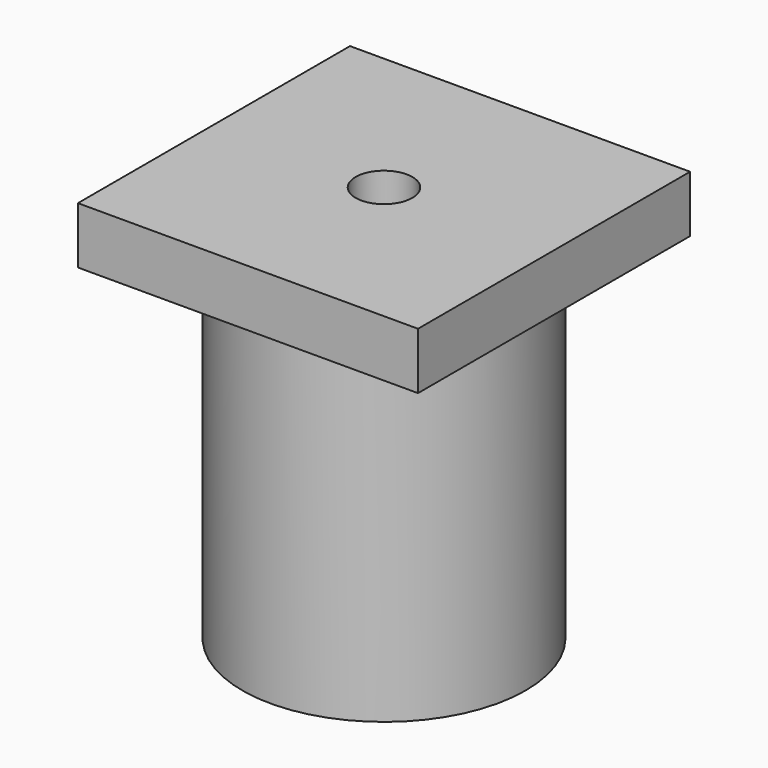
from build123d import *

# Parameters (mm, degrees)
F0_W     = 30
F0_H     = 30
F1_DEPTH = 35
F2_DEPTH = 30
F3_R     = 2.5
F4_DEPTH = 35.001
F5_W     = 30
F5_H     = 30
F5_R     = 12.5
F6_DEPTH = 30


with BuildPart() as f1:
    # F0 (on Top) → F1 (new body)
    with BuildSketch(Plane.XY):
        Rectangle(F0_W, F0_H)
        with BuildLine():
            ThreePointArc((-2.5, -6.5383484153), (-3.9686269666, 5.7662812973), (7, 0))
            ThreePointArc((7, 0), (5.7662812973, -3.9686269666), (2.5, -6.5383484153))
            Line((2.5, -6.5383484153), (2.5, -9.5))
            Line((2.5, -9.5), (0, -9.5))
            Line((0, -9.5), (-2.5, -9.5))
            Line((-2.5, -9.5), (-2.5, -6.5383484153))
        make_face(mode=Mode.SUBTRACT)
        with BuildLine():
            ThreePointArc((2.5, -6.5383484153), (5.7662812973, -3.9686269666), (7, 0))
            ThreePointArc((7, 0), (-3.9686269666, 5.7662812973), (-2.5, -6.5383484153))
            ThreePointArc((-2.5, -6.5383484153), (0, -7), (2.5, -6.5383484153))
        make_face()
        with BuildLine():
            ThreePointArc((2.5, -6.5383484153), (0, -7), (-2.5, -6.5383484153))
            Line((-2.5, -6.5383484153), (-2.5, -9.5))
            Line((-2.5, -9.5), (0, -9.5))
            Line((0, -9.5), (2.5, -9.5))
            Line((2.5, -9.5), (2.5, -6.5383484153))
        make_face()
    extrude(amount=F1_DEPTH)

    # F0 (on Top) → F2 (cut)
    with BuildSketch(Plane.XY):
        with BuildLine():
            ThreePointArc((2.5, -6.5383484153), (5.7662812973, -3.9686269666), (7, 0))
            ThreePointArc((7, 0), (-3.9686269666, 5.7662812973), (-2.5, -6.5383484153))
            ThreePointArc((-2.5, -6.5383484153), (0, -7), (2.5, -6.5383484153))
        make_face()
        with BuildLine():
            ThreePointArc((2.5, -6.5383484153), (0, -7), (-2.5, -6.5383484153))
            Line((-2.5, -6.5383484153), (-2.5, -9.5))
            Line((-2.5, -9.5), (0, -9.5))
            Line((0, -9.5), (2.5, -9.5))
            Line((2.5, -9.5), (2.5, -6.5383484153))
        make_face()
    extrude(amount=F2_DEPTH, mode=Mode.SUBTRACT)

    # F3 (on face) → F4 (cut, through all)
    with BuildSketch(Plane.XY.offset(35)):
        Circle(F3_R)
    extrude(amount=-F4_DEPTH, mode=Mode.SUBTRACT)

    # F5 (on face) → F6 (cut)
    with BuildSketch(Plane.XY):
        Rectangle(F5_W, F5_H)
        Circle(F5_R, mode=Mode.SUBTRACT)
    extrude(amount=F6_DEPTH, mode=Mode.SUBTRACT)


solid = f1.part
